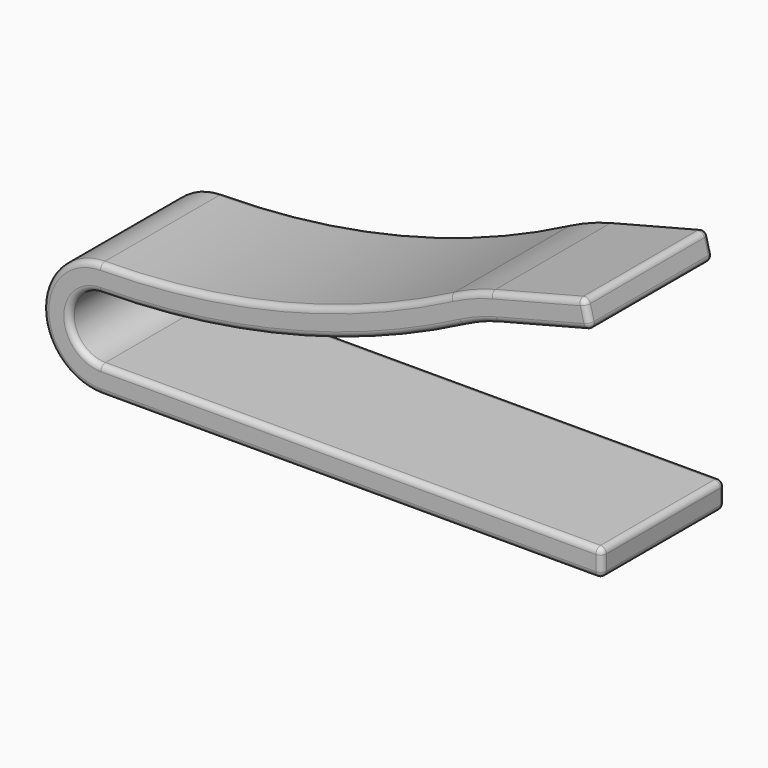
from build123d import *

# Parameters (mm, degrees)
F1_DEPTH = 20.32
F2_R     = 0.762


with BuildPart() as f1:
    # F0 (on Front) → F1 (new body)
    with BuildSketch(Plane.XZ):
        with BuildLine():
            Line((-32.2812777423, 0), (33.7587222577, 0))
            Line((33.7587222577, 0), (33.7587222577, 3.5))
            Line((33.7587222577, 3.5), (-32.2812777423, 3.5))
            ThreePointArc((-32.2812777423, 3.5), (-36.4012550506, 7.6063259449), (-32.308625702, 11.7399092331))
            ThreePointArc((-32.308625702, 11.7399092331), (-7.7452704082, 14.8185162016), (15.4165966965, 23.5571749303))
            ThreePointArc((15.4165966965, 23.5571749303), (17.6844448263, 24.575463703), (20.0530860269, 25.3301729364))
            Line((20.0530860269, 25.3301729364), (32.3530167072, 28.49272021))
            Line((32.3530167072, 28.49272021), (31.481448561, 31.8824648857))
            Line((31.481448561, 31.8824648857), (19.1815178806, 28.7199176121))
            ThreePointArc((19.1815178806, 28.7199176121), (16.4343267164, 27.8445927478), (13.8040371048, 26.6635637603))
            ThreePointArc((13.8040371048, 26.6635637603), (-8.5865023609, 18.215916502), (-32.331858192, 15.2398321253))
            ThreePointArc((-32.331858192, 15.2398321253), (-39.9012357736, 7.5947096359), (-32.2812777423, 0))
        make_face()
    extrude(amount=F1_DEPTH)

    # F2
    f2_edges = [f1.edges().sort_by_distance(p)[0] for p in [
        (16.434327, -20.32, 27.844593),
        (-8.586502, -20.32, 18.215917),
        (-39.901236, -20.32, 7.59471),
        (0.738722, -20.32, 0),
        (33.758722, -20.32, 1.75),
        (0.738722, -20.32, 3.5),
        (-36.401255, -20.32, 7.606326),
        (-7.74527, -20.32, 14.818516),
        (17.684445, -20.32, 24.575464),
        (26.203051, -20.32, 26.911447),
        (31.917233, -20.32, 30.187593),
        (25.331483, -20.32, 30.301191),
        (16.434327, 0, 27.844593),
        (-8.586502, 0, 18.215917),
        (-39.901236, 0, 7.59471),
        (0.738722, 0, 0),
        (33.758722, 0, 1.75),
        (0.738722, 0, 3.5),
        (-36.401255, 0, 7.606326),
        (-7.74527, 0, 14.818516),
        (17.684445, 0, 24.575464),
        (26.203051, 0, 26.911447),
        (31.917233, 0, 30.187593),
        (25.331483, 0, 30.301191),
        (32.353017, -10.16, 28.49272),
        (31.481449, -10.16, 31.882465),
        (33.758722, -10.16, 0),
        (33.758722, -10.16, 3.5),
    ]]
    fillet(f2_edges, radius=F2_R)


solid = f1.part
